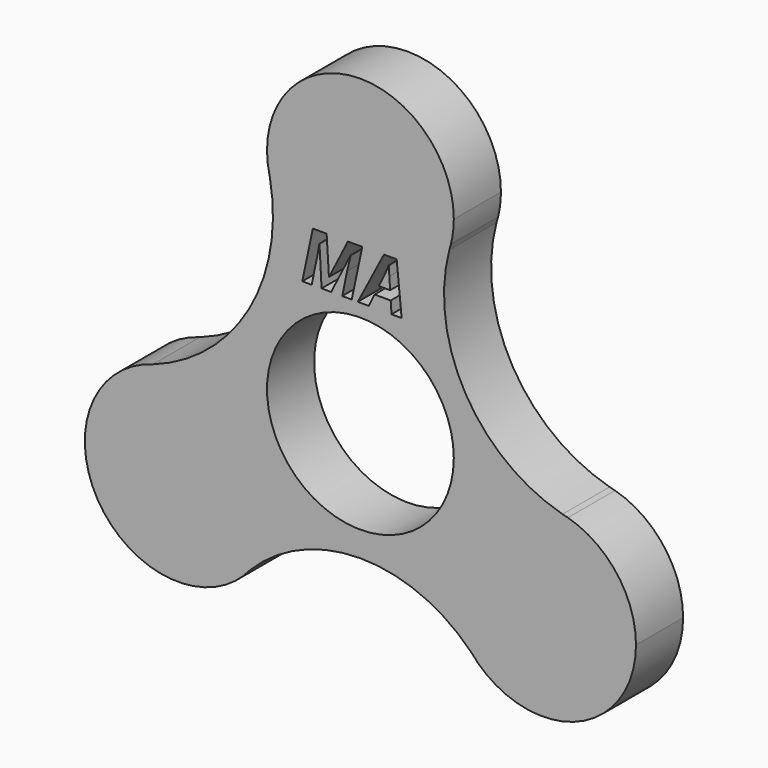
from build123d import *

# Parameters (mm, degrees)
F0_R         = 11.1
F1_DEPTH     = 7
F2_TEXT_SIZE = 8.3064401729
F3_DEPTH     = 7


# Not quite as in the source:
# - Text() gives the source's letters only with a copy of the font that has no kerning and outlines rounded to 1/6400 em; it was checked with that copy


with BuildPart() as f1:
    # F0 (on Front) → F1 (new body)
    with BuildSketch(Plane.XZ):
        with BuildLine():
            ThreePointArc((10.5768459141, 21.6324592788), (-0.3340251326, 13.9050269396), (-10.7602728632, 22.2748343338))
            ThreePointArc((-10.7602728632, 22.2748343338), (-13.2609230977, 7.6561975202), (-24.6707088297, -1.8187475157))
            ThreePointArc((-24.6707088297, -1.8187475157), (-14.9540993656, -3.6475196001), (-10.5506350946, -12.5))
            ThreePointArc((-10.5506350946, -12.5), (-11.2049874754, -16.2547897164), (-13.0908956017, -19.5668847319))
            ThreePointArc((-13.0908956017, -19.5668847319), (0, -14.0843518452), (13.0908956017, -19.5668847319))
            ThreePointArc((13.0908956017, -19.5668847319), (12.176030139, -6.7171061799), (24.0226822388, -1.6564123859))
            ThreePointArc((24.0226822388, -1.6564123859), (12.4846792181, 7.2080329073), (10.5768459141, 21.6324592788))
        make_face()
        Circle(F0_R, mode=Mode.SUBTRACT)
        with BuildLine():
            ThreePointArc((-10.5506350946, -12.5), (-14.9540993656, -3.6475196001), (-24.6707088297, -1.8187475157))
            ThreePointArc((-24.6707088297, -1.8187475157), (-31.2635170766, -18.05), (-13.9104359665, -20.4560868181))
            ThreePointArc((-13.9104359665, -20.4560868181), (-13.5079845537, -20.0047403713), (-13.0908956017, -19.5668847319))
            ThreePointArc((-13.0908956017, -19.5668847319), (-11.2049874754, -16.2547897164), (-10.5506350946, -12.5))
        make_face()
        with BuildLine():
            ThreePointArc((24.6707088297, -1.8187475157), (24.3459834367, -1.7404225776), (24.0226822388, -1.6564123859))
            ThreePointArc((24.0226822388, -1.6564123859), (12.176030139, -6.7171061799), (13.0908956017, -19.5668847319))
            ThreePointArc((13.0908956017, -19.5668847319), (13.5079845537, -20.0047403713), (13.9104359665, -20.4560868181))
            ThreePointArc((13.9104359665, -20.4560868181), (25.9688401429, -22.7256102586), (32.7506350946, -12.5))
            ThreePointArc((32.7506350946, -12.5), (30.5031154945, -5.803464271), (24.6707088297, -1.8187475157))
        make_face()
        with BuildLine():
            ThreePointArc((10.7602728632, 22.2748343338), (11.0147407773, 23.6268701413), (11.1, 25))
            ThreePointArc((11.1, 25), (-1.3731298587, 36.0147407773), (-10.7602728632, 22.2748343338))
            ThreePointArc((-10.7602728632, 22.2748343338), (-0.3340251326, 13.9050269396), (10.5768459141, 21.6324592788))
            ThreePointArc((10.5768459141, 21.6324592788), (10.6657415528, 21.9544514251), (10.7602728632, 22.2748343338))
        make_face()
    extrude(amount=F1_DEPTH)

    # F2 (on face) → F3 (cut)
    with BuildSketch(Plane.XZ.offset(7)):
        with Locations((-7.1223671548, 12.6430019736)):
            Text('MA', F2_TEXT_SIZE, font='Open Sans', font_style=FontStyle.BOLDITALIC, text_align=(TextAlign.LEFT, TextAlign.BOTTOM))
    extrude(amount=-F3_DEPTH, mode=Mode.SUBTRACT)


solid = f1.part
